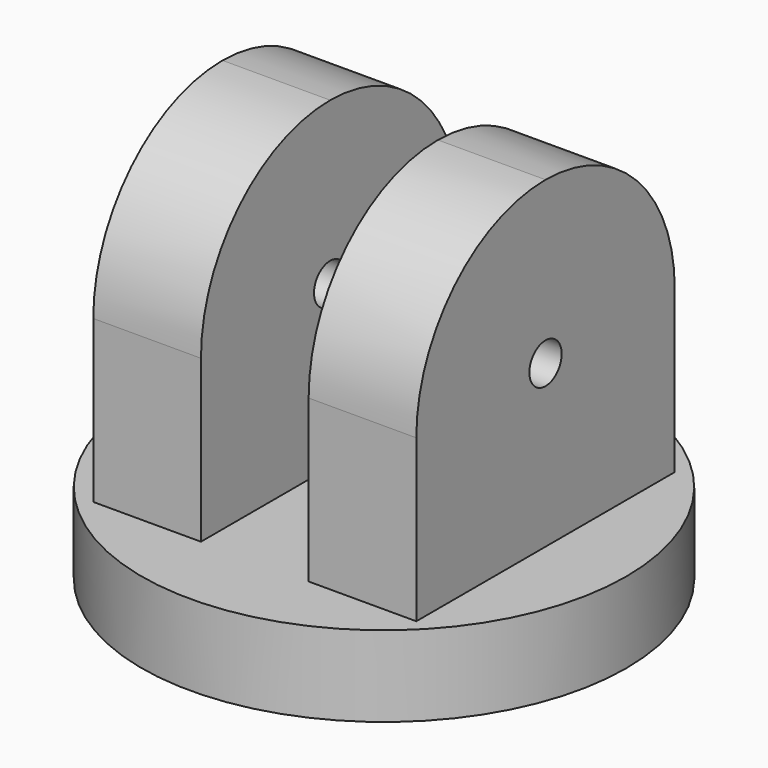
from build123d import *

# Parameters (mm, degrees)
F0_R     = 3.175
F1_DEPTH = 25.4
F0_R_2   = 38.1
F2_DEPTH = 12.7
F3_W     = 16.933164
F3_H     = 50.8
F3_W_2   = 16.933333164
F4_DEPTH = 50.8
F5_R     = 25.39999
F6_R     = 3.175
F7_DEPTH = 103.2441
F8_DEPTH = 120.64677


# Not quite as in the source:
# - a fillet or chamfer is up to 0.001 mm smaller than in the source, because OpenCascade refuses the exact size


with BuildPart() as f1:
    # F0 (on Top) → F1 (new body)
    with BuildSketch(Plane.XY):
        Circle(F0_R)
    extrude(amount=-F1_DEPTH)

    # F0 (on Top) → F2 (join)
    with BuildSketch(Plane.XY):
        Circle(F0_R_2)
        Circle(F0_R, mode=Mode.SUBTRACT)
        Circle(F0_R)
    extrude(amount=F2_DEPTH)

    # F3 (on face) → F4 (join)
    with BuildSketch(Plane.XY.offset(12.7)):
        with Locations((16.933418, 0)):
            Rectangle(F3_W, F3_H)
        with Locations((-16.933333418, 0)):
            Rectangle(F3_W_2, F3_H)
    extrude(amount=F4_DEPTH)

    # F5 (radius 25.4 in the source; OpenCascade refuses exactly that, so slightly less here)
    f5_edges = [f1.edges().sort_by_distance(p)[0] for p in [
        (16.933418, -25.4, 63.5),
        (16.933418, 25.4, 63.5),
        (-16.933333, 25.4, 63.5),
        (-16.933333, -25.4, 63.5),
    ]]
    fillet(f5_edges, radius=F5_R)

    # F6 (on face) → F7 (cut)
    with BuildSketch(Plane(origin=(-25.4, 0, 0), x_dir=(0, -1, 0), z_dir=(-1, 0, 0))):
        with Locations((0, 38.1)):
            Circle(F6_R)
    extrude(amount=-F7_DEPTH, mode=Mode.SUBTRACT)

    # F8 (cut): a face of the model
    f8_faces = [f1.faces().sort_by_distance(p)[0] for p in [
        (0, 0, -25.4),
    ]]
    extrude(f8_faces, amount=-F8_DEPTH, mode=Mode.SUBTRACT)


solid = f1.part
